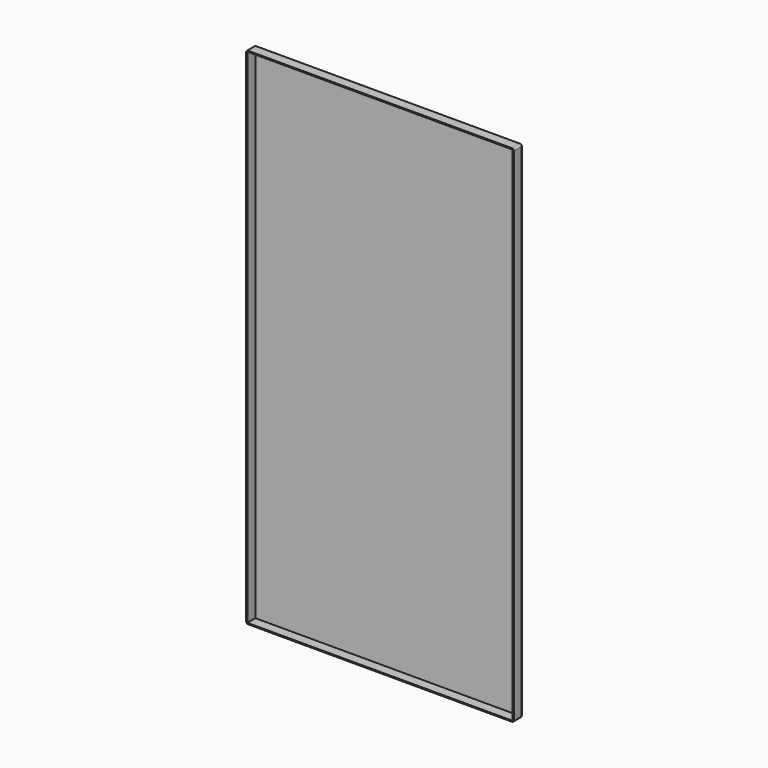
from build123d import *

# Parameters (mm, degrees)
F0_W         = 762
F0_H         = 1438.275
F1_DEPTH     = 3.175
F2_W         = 762
F2_H         = 1438.275
F2_W_2       = 755.65
F2_H_2       = 1431.925
F3_DEPTH     = 28.575
F4_R         = 5.08
F5_T1_DEPTH  = 39.37
F5_S5_W      = 5.1816
F5_S5_H      = 5.1816
F5_T6_DEPTH  = 5.1816
F5_S11_W     = 5.1816
F5_S11_H     = 5.1816
F5_T12_DEPTH = 5.1816
F5_S17_W     = 5.1816
F5_S17_H     = 5.1816
F5_T18_DEPTH = 5.1816
F5_S23_W     = 5.1816
F5_S23_H     = 5.1816
F5_T24_DEPTH = 5.1816


# Not quite as in the source:
# - a fillet or chamfer that OpenCascade refuses, or shapes differently, is made with other operations: its cross-section is extruded or revolved along the edge and cut away or added


with BuildPart() as f1:
    # F0 (on Front) → F1 (new body)
    with BuildSketch(Plane.XZ):
        Rectangle(F0_W, F0_H)
    extrude(amount=F1_DEPTH)

    # F2 (on face) → F3 (join)
    with BuildSketch(Plane.XZ.offset(3.175)):
        Rectangle(F2_W, F2_H)
        Rectangle(F2_W_2, F2_H_2, mode=Mode.SUBTRACT)
    extrude(amount=F3_DEPTH)

    # F4
    f4_edges = [f1.edges().sort_by_distance(p)[0] for p in [
        (0, 0, -719.1375),
        (381, 0, 0),
        (-381, 0, 0),
        (0, 0, 719.1375),
    ]]
    fillet(f4_edges, radius=F4_R)

    # F5: fillet of radius 5.08 on 4 edges, made by hand

    # F5_s2 → F5_t1 (cut)
    with BuildSketch(Plane.XZ.offset(5.08)):
        with BuildLine():
            ThreePointArc((-381, 714.0575), (-379.5121024484, 717.6496024484), (-375.92, 719.1375))
            Line((-375.92, 719.1375), (-381, 719.1375))
            Line((-381, 719.1375), (-381, 714.0575))
        make_face()
        with BuildLine():
            ThreePointArc((375.92, 719.1375), (379.5121024484, 717.6496024484), (381, 714.0575))
            Line((381, 714.0575), (381, 719.1375))
            Line((381, 719.1375), (375.92, 719.1375))
        make_face()
        with BuildLine():
            ThreePointArc((375.92, -719.1375), (379.5121024484, -717.6496024484), (381, -714.0575))
            Line((381, -714.0575), (381, -719.1375))
            Line((381, -719.1375), (375.92, -719.1375))
        make_face()
        with BuildLine():
            ThreePointArc((-381, -714.0575), (-379.5121024484, -717.6496024484), (-375.92, -719.1375))
            Line((-375.92, -719.1375), (-381, -719.1375))
            Line((-381, -719.1375), (-381, -714.0575))
        make_face()
    extrude(amount=F5_T1_DEPTH, mode=Mode.SUBTRACT)


with BuildPart() as f5_tool4:
    # F5_s5 → F5_t6 (new body)
    with BuildSketch(Plane.YZ.offset(-375.92)):
        with Locations((-2.4892, -716.6483)):
            Rectangle(F5_S5_W, F5_S5_H)
    extrude(amount=-F5_T6_DEPTH)

    # F5_s7 → F5_t8 (revolve, cut)
    with BuildSketch(Plane(origin=(-375.92, -5.08, -714.0575), x_dir=(0, -0.7071067812, 0.7071067812), z_dir=(0, -0.7071067812, -0.7071067812))):
        with BuildLine():
            ThreePointArc((0, -5.08), (5.08, 0), (0, 5.08))
            Line((0, 5.08), (0, -5.08))
        make_face()
    revolve(axis=Axis((-375.92, -5.08, -714.0575), (-1, 0, 0)), mode=Mode.SUBTRACT)


with BuildPart() as f1_1:
    add(f1.part)

    # F5_t3: cut F5_tool4
    add(f5_tool4.part, mode=Mode.SUBTRACT)


with BuildPart() as f5_tool10:
    # F5_s11 → F5_t12 (new body)
    with BuildSketch(Plane.XY.offset(-714.0575)):
        with Locations((378.5108, -2.4892)):
            Rectangle(F5_S11_W, F5_S11_H)
    extrude(amount=-F5_T12_DEPTH)

    # F5_s13 → F5_t14 (revolve, cut)
    with BuildSketch(Plane(origin=(375.92, -5.08, -714.0575), x_dir=(-0.7071067812, -0.7071067812, 0), z_dir=(0.7071067812, -0.7071067812, 0))):
        with BuildLine():
            ThreePointArc((0, -5.08), (5.08, 0), (0, 5.08))
            Line((0, 5.08), (0, -5.08))
        make_face()
    revolve(axis=Axis((375.92, -5.08, -714.0575), (0, 0, -1)), mode=Mode.SUBTRACT)


with BuildPart() as f1_2:
    add(f1_1.part)

    # F5_t9: cut F5_tool10
    add(f5_tool10.part, mode=Mode.SUBTRACT)


with BuildPart() as f5_tool16:
    # F5_s17 → F5_t18 (new body)
    with BuildSketch(Plane.XY.offset(714.0575)):
        with Locations((378.5108, -2.4892)):
            Rectangle(F5_S17_W, F5_S17_H)
    extrude(amount=F5_T18_DEPTH)

    # F5_s19 → F5_t20 (revolve, cut)
    with BuildSketch(Plane(origin=(375.92, -5.08, 714.0575), x_dir=(-0.7071067812, -0.7071067812, 0), z_dir=(-0.7071067812, 0.7071067812, 0))):
        with BuildLine():
            ThreePointArc((0, -5.08), (5.08, 0), (0, 5.08))
            Line((0, 5.08), (0, -5.08))
        make_face()
    revolve(axis=Axis((375.92, -5.08, 714.0575), (0, 0, 1)), mode=Mode.SUBTRACT)


with BuildPart() as f1_3:
    add(f1_2.part)

    # F5_t15: cut F5_tool16
    add(f5_tool16.part, mode=Mode.SUBTRACT)


with BuildPart() as f5_tool22:
    # F5_s23 → F5_t24 (new body)
    with BuildSketch(Plane.YZ.offset(-375.92)):
        with Locations((-2.4892, 716.6483)):
            Rectangle(F5_S23_W, F5_S23_H)
    extrude(amount=-F5_T24_DEPTH)

    # F5_s25 → F5_t26 (revolve, cut)
    with BuildSketch(Plane(origin=(-375.92, -5.08, 714.0575), x_dir=(0, -0.7071067812, -0.7071067812), z_dir=(0, 0.7071067812, -0.7071067812))):
        with BuildLine():
            ThreePointArc((0, -5.08), (5.08, 0), (0, 5.08))
            Line((0, 5.08), (0, -5.08))
        make_face()
    revolve(axis=Axis((-375.92, -5.08, 714.0575), (-1, 0, 0)), mode=Mode.SUBTRACT)


with BuildPart() as f1_4:
    add(f1_3.part)

    # F5_t21: cut F5_tool22
    add(f5_tool22.part, mode=Mode.SUBTRACT)


solid = f1_4.part
